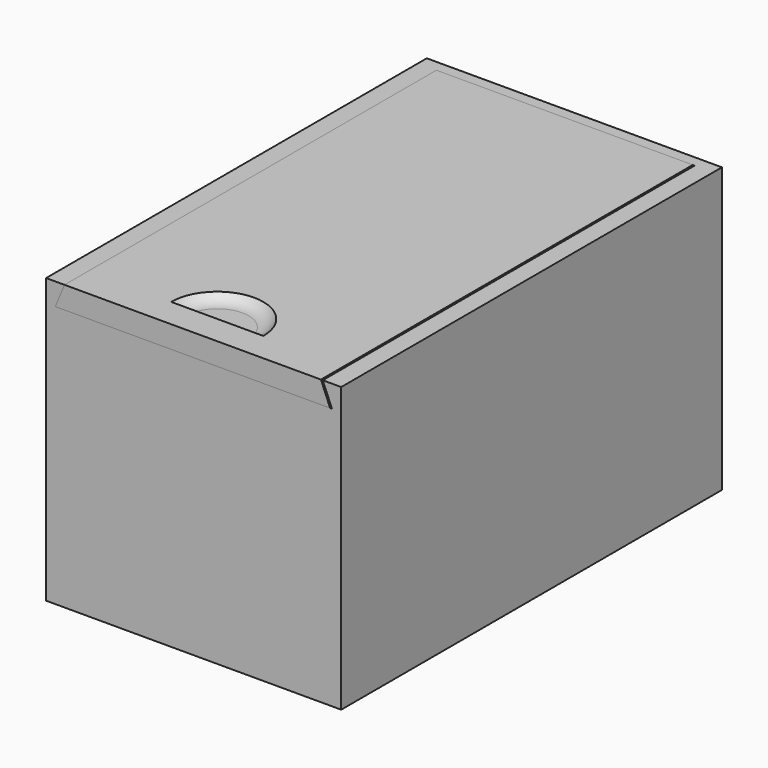
from build123d import *

# Parameters (mm, degrees)
F0_W         = 76
F0_H         = 99
F0_W_2       = 70
F0_H_2       = 93
F1_DEPTH     = 77
F2_T         = -3
F3_DEPTH     = 30
F4_T         = -3
F5_DEPTH     = 2
F6_DEPTH     = 2
F8_DEPTH     = 126
F10_DEPTH    = 126
F12_DEPTH    = 2
F13_T2_ANGLE = 180


# Not quite as in the source:
# - a fillet or chamfer that OpenCascade refuses, or shapes differently, is made with other operations: its cross-section is extruded or revolved along the edge and cut away or added


with BuildPart() as f1:
    # F0 (on Top) → F1 (new body)
    with BuildSketch(Plane.XY):
        with Locations((35, -46.5)):
            Rectangle(F0_W, F0_H)
        with Locations((35, -46.5)):
            Rectangle(F0_W_2, F0_H_2, mode=Mode.SUBTRACT)
        with Locations((35, -46.5)):
            Rectangle(F0_W_2, F0_H_2)
    extrude(amount=F1_DEPTH)

    # F2
    f2_openings = [f1.faces().sort_by_distance(p)[0] for p in [
        (35, -46.5, 77),
    ]]
    offset(amount=F2_T, openings=f2_openings)

    # F3 (add): a face of the model
    f3_faces = [f1.faces().sort_by_distance(p)[0] for p in [
        (35, 3, 38.5),
    ]]
    extrude(f3_faces, amount=F3_DEPTH)

    # F4: a shell. OpenCascade refuses it in one call, so the cavity is built on its own and cut out:
    # the body offset inwards by the wall thickness, plus a prism from it out through each open face.
    f4_core = offset(f1.part, amount=F4_T, kind=Kind.INTERSECTION, mode=Mode.PRIVATE)
    f4_exits = [f4_core.faces().sort_by_distance(p)[0] for p in [
        (35, 16.5, 74),
    ]]
    add(f4_core, mode=Mode.SUBTRACT)
    extrude(f4_exits, amount=-F4_T, mode=Mode.SUBTRACT)

    # F5 (add): a face of the model
    f5_faces = [f1.faces().sort_by_distance(p)[0] for p in [
        (-3, -31.5, 38.5),
    ]]
    extrude(f5_faces, amount=F5_DEPTH)

    # F6 (add): a face of the model
    f6_faces = [f1.faces().sort_by_distance(p)[0] for p in [
        (73, -31.5, 38.5),
    ]]
    extrude(f6_faces, amount=F6_DEPTH)

    # F7 (on face) → F8 (cut, through all)
    with BuildSketch(Plane.XZ.offset(96)):
        Polygon((70, 77), (0, 77), (-2.5, 71), (72.5, 71), align=None)
    extrude(amount=-F8_DEPTH, mode=Mode.SUBTRACT)


with BuildPart() as f10:
    # F9 (on face) → F10 (new body, through all)
    with BuildSketch(Plane.XZ.offset(96)):
        Polygon((69.5, 77), (0, 77), (-2.5, 71), (72, 71), align=None)
    extrude(amount=-F10_DEPTH)

    # F11 (on face) → F12 (cut)
    with BuildSketch(Plane.XY.offset(77)):
        with BuildLine():
            Line((22.5, -88), (47.5, -88))
            ThreePointArc((47.5, -88), (35, -75.5), (22.5, -88))
        make_face()
    extrude(amount=-F12_DEPTH, mode=Mode.SUBTRACT)

    # F13: fillet of radius 5 on 1 edges, made by hand

    # F13_s1 → F13_t2 (revolve)
    with BuildSketch(Plane.XZ.offset(88)):
        with BuildLine():
            ThreePointArc((47.5, 77), (45.7360679775, 75.527864045), (43.5, 75))
            Line((43.5, 75), (47.5, 75))
            Line((47.5, 75), (47.5, 77))
        make_face()
    revolve(axis=Axis((35, -88, 75), (0, 0, 1)), revolution_arc=F13_T2_ANGLE)


solid = Compound([f1.part, f10.part])
